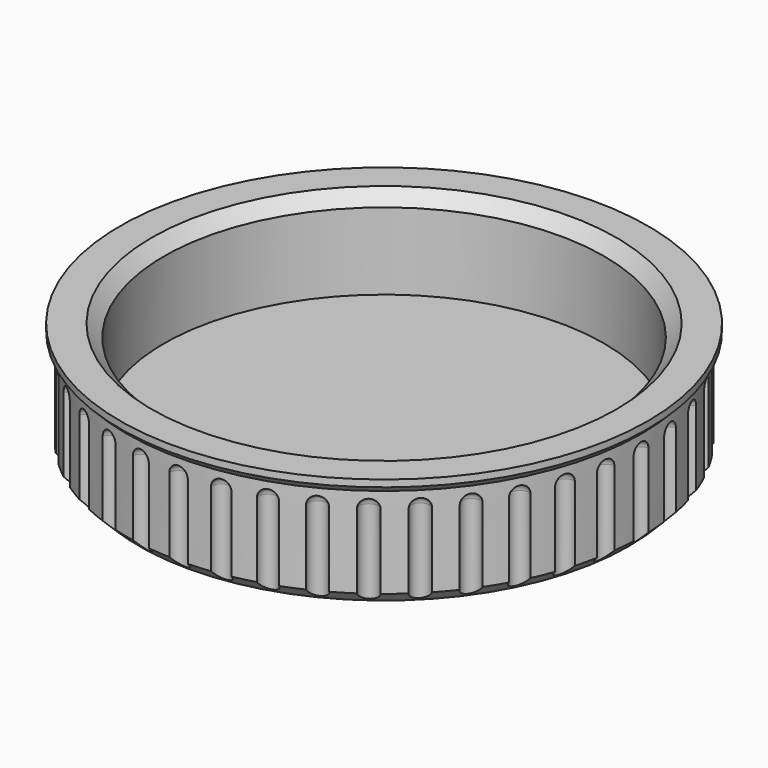
from build123d import *

# Parameters (mm, degrees)
F1_R            = 18.75
F1_R_2          = 16.05
F2_DEPTH        = 8.5
F3_DEPTH        = 2
F4_SIZE         = 0.9
F6_COPIES_COUNT = 40


# Not quite as in the source:
# - two fillets or chamfers of one size are made in one step
# - a pattern or mirror of a feature is missing from the dataset's text; its kind, count and spacing are read off the source's solid


with BuildPart() as f2:
    # F1 (on Top) → F2 (new body)
    with BuildSketch(Plane.XY):
        Circle(F1_R)
        Circle(F1_R_2, mode=Mode.SUBTRACT)
    extrude(amount=F2_DEPTH)

    # F1 (on Top) → F3 (join)
    with BuildSketch(Plane.XY):
        Circle(F1_R_2)
    extrude(amount=F3_DEPTH)

    # F4
    f4_edges = [f2.edges().sort_by_distance(p)[0] for p in [
        (-18.75, 0, 0),
        (-16.05, 0, 8.5),
    ]]
    chamfer(f4_edges, length=F4_SIZE)

    # F5 (on Front) → F6 (revolve, cut)
    with BuildSketch(Plane.XZ):
        with BuildLine():
            Line((18.075, 6.325), (18.075, 0))
            Line((18.075, 0), (18.75, 0))
            Line((18.75, 0), (18.75, 7))
            ThreePointArc((18.75, 7), (18.2727029227, 6.8022970773), (18.075, 6.325))
        make_face()
    f6 = revolve(axis=Axis((18.75, 0, 3.5), (0, 0, -1)), mode=Mode.SUBTRACT)

    # F6_copies: F6 ×40 about axis
    f6_copies_axis = Axis((0, 0, 0), (0, 0, 1))
    for i in range(1, F6_COPIES_COUNT):
        add(f6.rotate(f6_copies_axis, i * 360 / F6_COPIES_COUNT), mode=Mode.SUBTRACT)

    # F7 (on Front) → F8 (revolve)
    with BuildSketch(Plane.XZ):
        Polygon((19.25, 8.5), (18.75, 8.5), (18.75, 7.5), (19.25, 8), align=None)
    revolve(axis=Axis((0, 0, 8.5), (0, 0, 1)))


solid = f2.part
